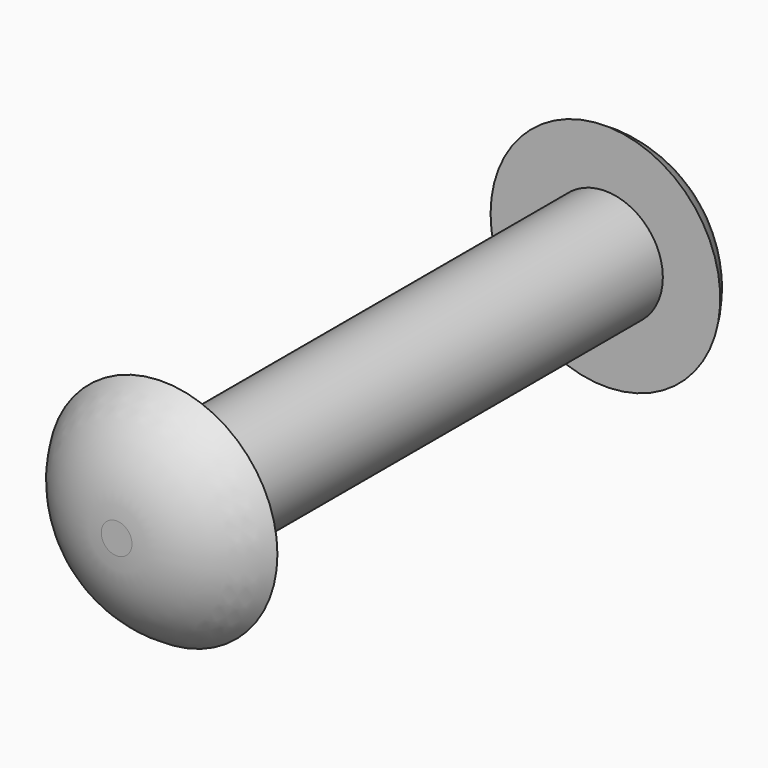
from build123d import *

# Parameters (mm, degrees)
F0_R     = 0.5
F1_DEPTH = 2.41
F2_R     = 1
F3_DEPTH = 0.5
F4_R     = 1
F5_DEPTH = 0.5


# Not quite as in the source:
# - a fillet or chamfer that OpenCascade refuses, or shapes differently, is made with other operations: its cross-section is extruded or revolved along the edge and cut away or added


with BuildPart() as f1:
    # F0 (on Front) → F1 (new body, symmetric)
    with BuildSketch(Plane.XZ):
        Circle(F0_R)
    extrude(amount=F1_DEPTH, both=True)

    # F2 (on face) → F3 (join)
    with BuildSketch(Plane.XZ.offset(2.41)):
        Circle(F2_R)
    extrude(amount=F3_DEPTH)

    # F4 (on face) → F5 (join)
    with BuildSketch(Plane(origin=(0, 2.41, 0), x_dir=(-1, 0, 0), z_dir=(0, 1, 0))):
        Circle(F4_R)
    extrude(amount=F5_DEPTH)

    # F6: fillet of radius 1 on 2 edges, made by hand

    # F6_s1 → F6_t2 (revolve, cut)
    with BuildSketch(Plane.XY):
        with BuildLine():
            ThreePointArc((-1, 2.41), (-0.6339745962, 2.7760254038), (-0.1339745962, 2.91))
            Line((-0.1339745962, 2.91), (-1, 2.91))
            Line((-1, 2.91), (-1, 2.41))
        make_face()
    revolve(axis=Axis((0, 2.91, 0), (0, 1, 0)), mode=Mode.SUBTRACT)

    # F6_s3 → F6_t4 (revolve, cut)
    with BuildSketch(Plane.XY):
        with BuildLine():
            ThreePointArc((1, -2.41), (0.6339745962, -2.7760254038), (0.1339745962, -2.91))
            Line((0.1339745962, -2.91), (1, -2.91))
            Line((1, -2.91), (1, -2.41))
        make_face()
    revolve(axis=Axis((0, -2.91, 0), (0, -1, 0)), mode=Mode.SUBTRACT)


solid = f1.part
